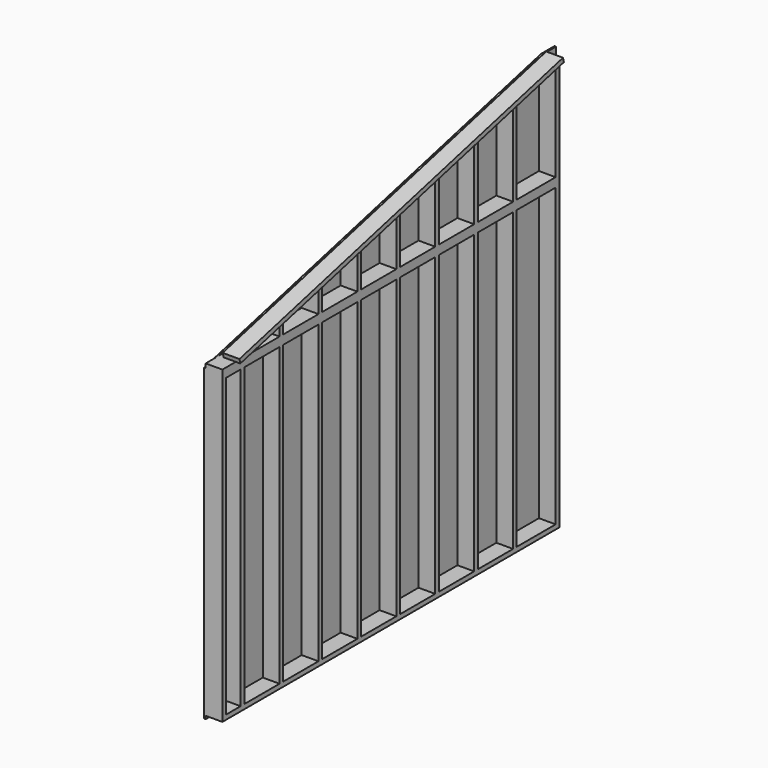
from build123d import *

# Parameters (mm, degrees)
F0_W      = 139.7
F0_H      = 3517.9
F1_DEPTH  = 38.1
F3_DEPTH  = 139.7
F4_W      = 139.7
F4_H      = 38.1
F5_REACH  = 3576.7609868968
F6_W      = 38.1
F6_H      = 3481.6151260149
F7_DEPTH  = 38.1
F9_DEPTH  = 38.1
F11_DEPTH = 12.7


with BuildPart() as f1:
    # F0 (on Top) → F1 (new body)
    with BuildSketch(Plane.XY):
        Rectangle(F0_W, F0_H)
    extrude(amount=F1_DEPTH)

    # F2 (on face) → F3 (join, through all)
    with BuildSketch(Plane.YZ.offset(69.85)):
        Polygon((1720.85, 2590.8), (-1758.95, 2590.8), (-1758.95, 38.1), (-1720.85, 38.1), (-1720.85, 2514.6), (1720.85, 2514.6), (1720.85, 38.1), (1758.95, 38.1), (1758.95, 2590.8), (1758.95, 3433.0894), (1749.7329391709, 3470.0577079092), (-1628.4670608291, 2627.7937079092), (-1619.25, 2590.8254), (1720.85, 3423.5901819549), align=None)
    extrude(amount=-F3_DEPTH)

    f5_end = f1.faces().sort_by_distance((0, 50.8, 3007.2077909774))[0]
    # F4 (on face) → F5 (join, up to a face of the model that its end follows)
    with BuildSketch(Plane.XY.offset(38.1)):
        with Locations((0, 1295.4)):
            Rectangle(F4_W, F4_H)
        with Locations((0, 889)):
            Rectangle(F4_W, F4_H)
        with Locations((0, 482.6)):
            Rectangle(F4_W, F4_H)
        with Locations((0, 76.2)):
            Rectangle(F4_W, F4_H)
        with Locations((0, -330.2)):
            Rectangle(F4_W, F4_H)
        with Locations((0, -736.6)):
            Rectangle(F4_W, F4_H)
        with Locations((0, -1143)):
            Rectangle(F4_W, F4_H)
        with Locations((0, -1549.4)):
            Rectangle(F4_W, F4_H)
    f5_long = extrude(amount=F5_REACH, mode=Mode.PRIVATE)
    add(split(f5_long, bisect_by=f5_end, keep=Keep.TOP, mode=Mode.PRIVATE))

    # F6 (on face) → F7 (cut)
    with BuildSketch(Plane(origin=(0, -712.1315701529, 2856.2575039305), x_dir=(1, 0, 0), z_dir=(0, -0.2419176071, 0.9702967955))):
        with Locations((-50.8, 796.4207579507)):
            Rectangle(F6_W, F6_H)
    extrude(amount=-F7_DEPTH, mode=Mode.SUBTRACT)

    # F8 (on face) → F9 (join)
    with BuildSketch(Plane.YZ.offset(69.85)):
        Polygon((1749.7329391709, 3470.0577079092), (-1628.4670608291, 2627.7937079092), (-1619.25, 2590.8254), (1758.95, 3433.0894), align=None)
    extrude(amount=F9_DEPTH)

    # F10 (on face) → F11 (join)
    with BuildSketch(Plane(origin=(-69.85, 0, 0), x_dir=(0, -1, 0), z_dir=(-1, 0, 0))):
        Polygon((-1898.65, -25.4), (1758.95, -25.4), (1758.95, 2555.9949338346), (-1758.95, 3433.0894), (-1898.65, 3433.0894), (-1898.65, 0), align=None)
    extrude(amount=F11_DEPTH)


solid = f1.part
